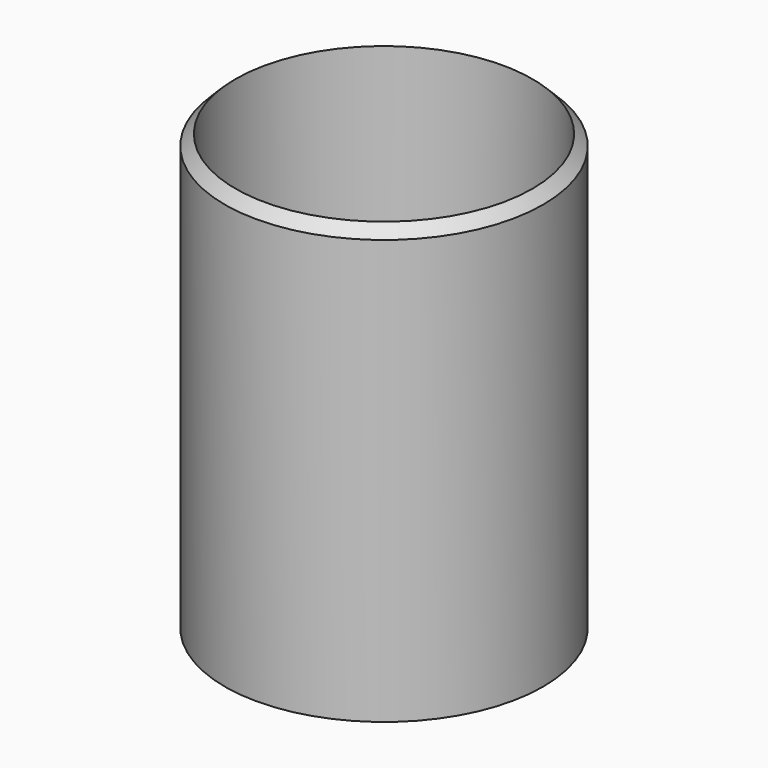
from build123d import *

# Parameters (mm, degrees)
F0_R     = 37.5
F1_DEPTH = 105
F2_R     = 35
F3_DEPTH = 100


# Not quite as in the source:
# - a fillet or chamfer that OpenCascade refuses, or shapes differently, is made with other operations: its cross-section is extruded or revolved along the edge and cut away or added


with BuildPart() as f1:
    # F0 (on Top) → F1 (new body)
    with BuildSketch(Plane.XY):
        Circle(F0_R)
    extrude(amount=F1_DEPTH)

    # F2 (on face) → F3 (cut)
    with BuildSketch(Plane.XY.offset(105)):
        Circle(F2_R)
    extrude(amount=-F3_DEPTH, mode=Mode.SUBTRACT)

    # F4: chamfer of 5 on 1 edges, made by hand

    # F4_s1 → F4_t2 (revolve, cut)
    with BuildSketch(Plane.XZ):
        Polygon((37.5, 100), (32.5, 105), (37.5, 105), align=None)
    revolve(axis=Axis((0, 0, 105), (0, 0, 1)), mode=Mode.SUBTRACT)


solid = f1.part
